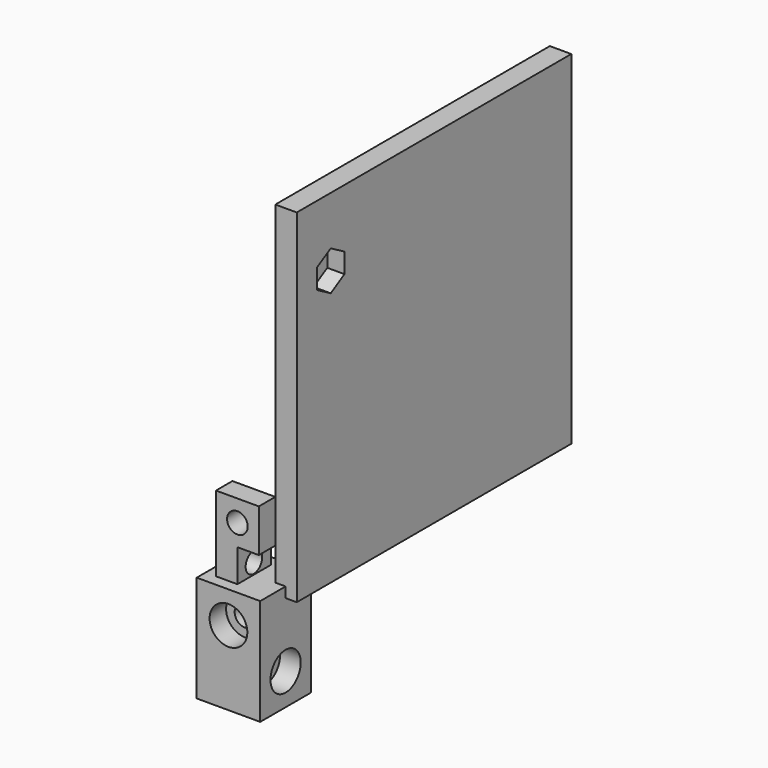
from build123d import *

# Parameters (mm, degrees)
F0_W          = 12.5
F0_H          = 25
F0_R          = 3
F1_DEPTH      = 6
F3_START      = -6.25
F2_W          = 6.25
F2_H          = 12.5
F3_DEPTH      = 6.25
F4_W          = 6.25
F4_H          = 12.5
F5_DEPTH      = 25
F6_R          = 3
F7_DEPTH      = 25
F8_W          = 12.5
F8_H          = 25
F9_DEPTH      = 6.25
F9_DEPTH_BACK = 6.25
F10_R         = 3
F11_DEPTH     = 25
F12_R         = 3
F13_DEPTH     = 25
F14_DEPTH     = 3
F15_DEPTH     = 3
F16_DEPTH     = 3
F17_DEPTH     = 3
F18_DEPTH     = 3
F19_DEPTH     = 3
F20_R         = 5.5
F20_R_2       = 3
F21_DEPTH     = 6
F22_R         = 5.5
F22_R_2       = 3
F23_DEPTH     = 6
F24_W         = 100
F24_H         = 100
F25_DEPTH     = 6.25
F27_DEPTH     = 5


with BuildPart() as f1:
    # F0 (on Front) → F1 (new body)
    with BuildSketch(Plane.XZ):
        with Locations((-6.25, 12.5)):
            Rectangle(F0_W, F0_H)
        with Locations((-6.25, 18.75)):
            Circle(F0_R, mode=Mode.SUBTRACT)
    extrude(amount=F1_DEPTH)

    # F2 (on Right) → F3 (join)
    with BuildSketch(Plane.YZ.offset(F3_START)):
        with Locations((3.125, 6.25)):
            Rectangle(F2_W, F2_H)
    extrude(amount=-F3_DEPTH)

    # F4 (on face) → F5 (cut)
    with BuildSketch(Plane(origin=(0, 0, 0), x_dir=(-1, 0, 0), z_dir=(0, 1, 0))):
        with Locations((3.125, 6.25)):
            Rectangle(F4_W, F4_H)
    extrude(amount=-F5_DEPTH, mode=Mode.SUBTRACT)

    # F6 (on face) → F7 (cut)
    with BuildSketch(Plane.YZ.offset(-6.25)):
        with Locations((0, 6.25)):
            Circle(F6_R)
    extrude(amount=-F7_DEPTH, mode=Mode.SUBTRACT)


with BuildPart() as f9:
    # F8 (on Front) → F9 (new body, two sides)
    with BuildSketch(Plane.XZ) as f9_sk:
        with Locations((-6.25, -12.5)):
            Rectangle(F8_W, F8_H)
    extrude(amount=-F9_DEPTH)
    extrude(f9_sk.sketch, amount=F9_DEPTH_BACK)

    # F10 (on face) → F11 (cut)
    with BuildSketch(Plane(origin=(0, 6.25, 0), x_dir=(-1, 0, 0), z_dir=(0, 1, 0))):
        with Locations((6.25, -6.25)):
            Circle(F10_R)
    extrude(amount=-F11_DEPTH, mode=Mode.SUBTRACT)

    # F12 (on face) → F13 (cut)
    with BuildSketch(Plane.YZ):
        with Locations((0, -18.75)):
            Circle(F12_R)
    extrude(amount=-F13_DEPTH, mode=Mode.SUBTRACT)

    # F14 (add): a face of the model
    f14_faces = [f9.faces().sort_by_distance(p)[0] for p in [
        (-6.25, -6.25, -13.1217404261),
    ]]
    extrude(f14_faces, amount=F14_DEPTH)

    # F15 (add): a face of the model
    f15_faces = [f9.faces().sort_by_distance(p)[0] for p in [
        (-6.25, 6.25, -13.1217404261),
    ]]
    extrude(f15_faces, amount=F15_DEPTH)

    # F16 (add): a face of the model
    f16_faces = [f9.faces().sort_by_distance(p)[0] for p in [
        (0, 0, -12.0930351415),
    ]]
    extrude(f16_faces, amount=F16_DEPTH)

    # F17 (add): a face of the model
    f17_faces = [f9.faces().sort_by_distance(p)[0] for p in [
        (-12.5, 0, -12.0930351415),
    ]]
    extrude(f17_faces, amount=F17_DEPTH)

    # F18 (add): a face of the model
    f18_faces = [f9.faces().sort_by_distance(p)[0] for p in [
        (-6.25, 0, 0),
    ]]
    extrude(f18_faces, amount=F18_DEPTH)

    # F19 (add): a face of the model
    f19_faces = [f9.faces().sort_by_distance(p)[0] for p in [
        (-6.25, 0, -25),
    ]]
    extrude(f19_faces, amount=F19_DEPTH)

    # F20 (on face) → F21 (cut)
    with BuildSketch(Plane.YZ.offset(3)):
        with Locations((0, -18.75)):
            Circle(F20_R)
        with Locations((0, -18.75)):
            Circle(F20_R_2, mode=Mode.SUBTRACT)
    extrude(amount=-F21_DEPTH, mode=Mode.SUBTRACT)

    # F22 (on face) → F23 (cut)
    with BuildSketch(Plane.XZ.offset(9.25)):
        with Locations((-6.25, -6.25)):
            Circle(F22_R)
        with Locations((-6.25, -6.25)):
            Circle(F22_R_2, mode=Mode.SUBTRACT)
    extrude(amount=-F23_DEPTH, mode=Mode.SUBTRACT)


with BuildPart() as f25:
    # F24 (on Right) → F25 (new body)
    with BuildSketch(Plane.YZ):
        with Locations((50, 50)):
            Rectangle(F24_W, F24_H)
    extrude(amount=F25_DEPTH)

    # F26 (on face) → F27 (cut)
    with BuildSketch(Plane.YZ.offset(6.25)):
        Polygon((12.375, 74.2264973081), (17.375, 77.1132486541), (17.375, 82.8867513459), (12.375, 85.7735026919), (7.375, 82.8867513459), (7.375, 77.1132486541), align=None)
    extrude(amount=-F27_DEPTH, mode=Mode.SUBTRACT)


solid = Compound([f1.part, f9.part, f25.part])
